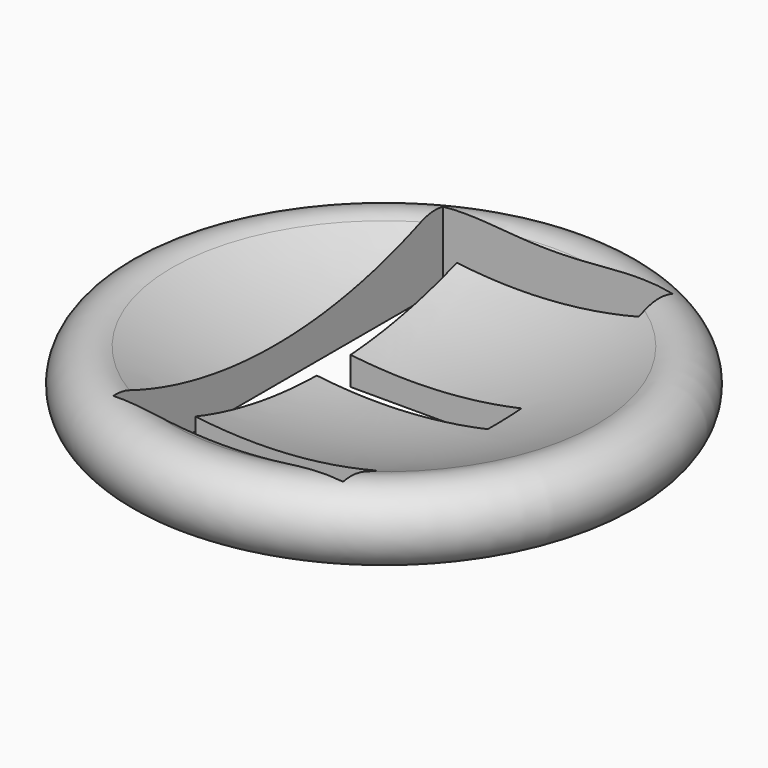
from build123d import *

# Parameters (mm, degrees)
F2_TEXT_SIZE = 141.1111111111
F3_DEPTH     = 25.4


# Not quite as in the source:
# - Text() gives the source's letters only with a copy of the font that has no kerning and outlines rounded to 1/6400 em; it was checked with that copy


with BuildPart() as f1:
    # F0 (on Front) → F1 (revolve)
    with BuildSketch(Plane.XZ):
        with BuildLine():
            ThreePointArc((0, 5.7720580461), (-26.5516746187, 8.6193887324), (-51.8958744513, 17.0318944196))
            ThreePointArc((-51.8958744513, 17.0318944196), (-64.305370772, 10.8075371262), (-55.5912808072, 0))
            Line((-55.5912808072, 0), (0, 0))
            Line((0, 0), (0, 5.7720580461))
        make_face()
    revolve(axis=Axis((0, 0, 2.886029023), (0, 0, 1)))

    # F2 (on Top) → F3 (cut)
    with BuildSketch(Plane.XY):
        with Locations((-40.436730659, -49.4622857512)):
            Text('E', F2_TEXT_SIZE, font='Open Sans', text_align=(TextAlign.LEFT, TextAlign.BOTTOM))
    extrude(amount=F3_DEPTH, mode=Mode.SUBTRACT)


solid = f1.part
